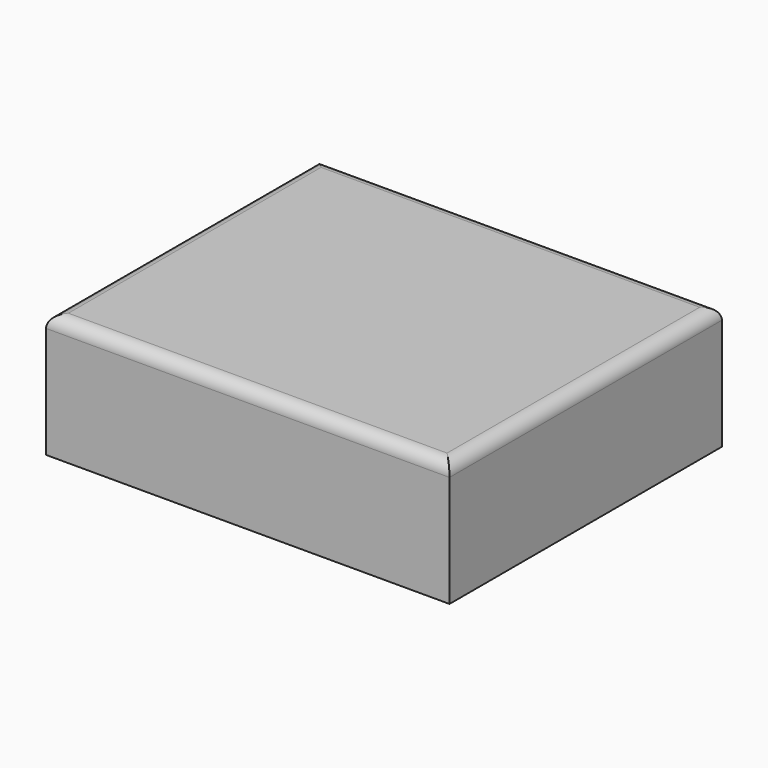
from build123d import *

# Parameters (mm, degrees)
F0_W     = 162.9769206047
F0_H     = 137.5593692064
F1_DEPTH = 50
F3_R     = 5


# Not quite as in the source:
# - a feature of the source that left no trace in its solid (it failed there, or was rolled back) is left out


with BuildPart() as f1:
    # F0 (on Top) → F1 (new body)
    with BuildSketch(Plane.XY):
        with Locations((7.5951814651, 5.6864470243)):
            Rectangle(F0_W, F0_H)
    extrude(amount=F1_DEPTH)

    # F3
    f3_edges = [f1.edges().sort_by_distance(p)[0] for p in [
        (89.083642, 5.686447, 50),
        (7.595181, -63.093238, 50),
        (-73.893279, 5.686447, 50),
        (7.595181, 74.466132, 50),
    ]]
    fillet(f3_edges, radius=F3_R)


solid = f1.part
